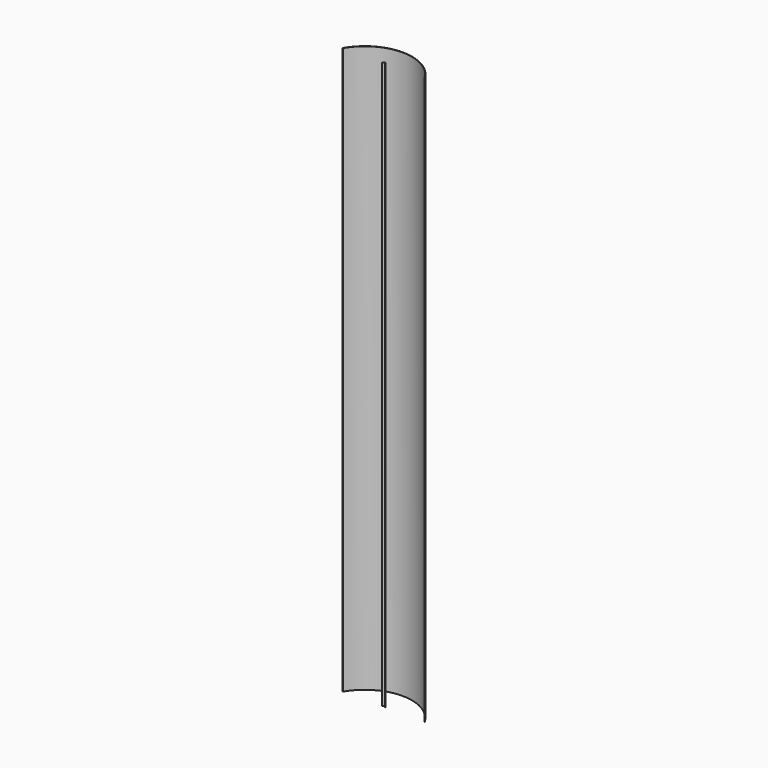
from build123d import *

# Parameters (mm, degrees)
F1_DEPTH = 3000
F2_DEPTH = 3000


with BuildPart() as f1:
    # F0 (on Top) → F1 (new body)
    with BuildSketch(Plane.XY):
        with BuildLine():
            ThreePointArc((-216.0716027154, 125.75), (0, 250), (216.0716027154, 125.75))
            Line((216.0716027154, 125.75), (217.8053890518, 125.75))
            ThreePointArc((217.8053890518, 125.75), (0, 251.5), (-217.8053890518, 125.75))
            Line((-217.8053890518, 125.75), (-216.0716027154, 125.75))
        make_face()
    extrude(amount=F1_DEPTH)


with BuildPart() as f2:
    # F0 (on Top) → F2 (new body)
    with BuildSketch(Plane.XY):
        with BuildLine():
            ThreePointArc((-216.0716027154, 125.75), (0, 250), (216.0716027154, 125.75))
            Line((216.0716027154, 125.75), (217.8053890518, 125.75))
            ThreePointArc((217.8053890518, 125.75), (0, 251.5), (-217.8053890518, 125.75))
            Line((-217.8053890518, 125.75), (-216.0716027154, 125.75))
        make_face()
    extrude(amount=F2_DEPTH)


with BuildPart() as f2b:
    # F0 (on Top) → F2, piece 2 (new body)
    with BuildSketch(Plane.XY):
        with BuildLine():
            ThreePointArc((-7.5, 125.75), (0, 133.25), (7.5, 125.75))
            Line((7.5, 125.75), (8.5, 125.75))
            ThreePointArc((8.5, 125.75), (0, 134.25), (-8.5, 125.75))
            Line((-8.5, 125.75), (-7.5, 125.75))
        make_face()
    extrude(amount=F2_DEPTH)


solid = Compound([f1.part, f2.part, f2b.part])
